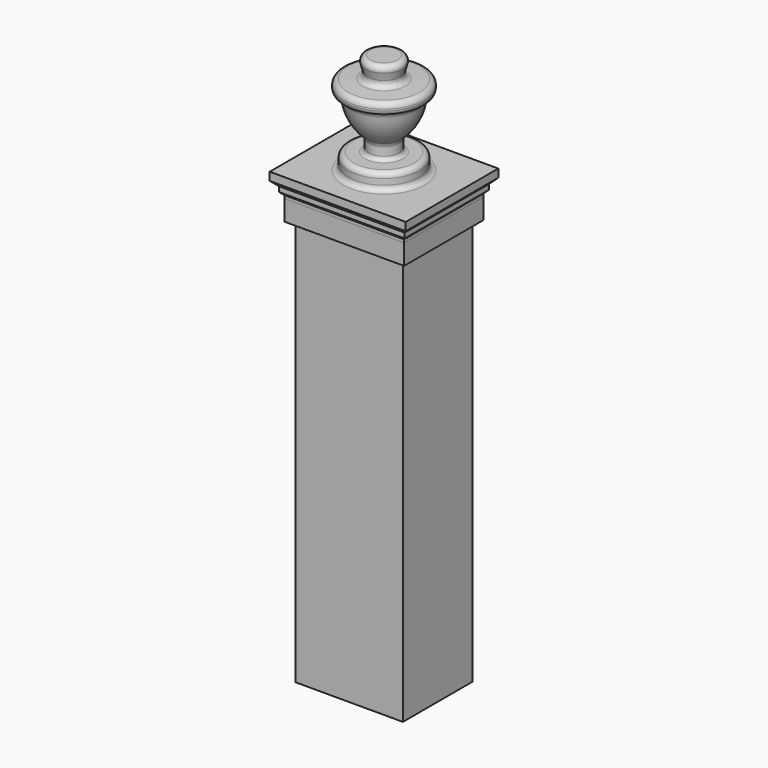
from build123d import *

# Parameters (mm, degrees)
F0_W     = 530
F0_H     = 430
F1_DEPTH = 2000
F2_W     = 590
F2_H     = 490
F3_DEPTH = 100
F6_W     = 510
F6_H     = 410
F7_DEPTH = 120
F10_R    = 25.4
F11_R    = 19.05


with BuildPart() as f1:
    # F0 (on Top) → F1 (new body)
    with BuildSketch(Plane.XY):
        Rectangle(F0_W, F0_H)
    extrude(amount=F1_DEPTH)

    # F2 (on face) → F3 (join)
    with BuildSketch(Plane.XY.offset(2000)):
        Rectangle(F2_W, F2_H)
    extrude(amount=F3_DEPTH)


with BuildPart() as f5:
    # F5: sweep along a path in F5_path
    with BuildLine(Plane(origin=(295, -245, 2100), x_dir=(0, 1, 0), z_dir=(0, 0, 1))) as f5_path:
        Line((0, 0), (0, 590))
        Line((0, 590), (490, 590))
        Line((490, 590), (490, 0))
        Line((490, 0), (0, 0))
    # F4 (on Right) → F5 (sweep)
    with BuildSketch(Plane.YZ):
        Polygon((-245, 2115), (-245, 2100), (-205, 2100), (-205, 2220), (-285, 2220), (-285, 2180), (-260, 2155), (-260, 2130), align=None)
    sweep(path=f5_path.line, transition=Transition.RIGHT)

    # F6 (on face) → F7 (join, through all)
    with BuildSketch(Plane.XY.offset(2220)):
        Rectangle(F6_W, F6_H)
    extrude(amount=-F7_DEPTH)

    # F8 (on Right) → F9 (revolve)
    with BuildSketch(Plane.YZ):
        with BuildLine():
            Line((100, 2720), (0, 2720))
            Line((0, 2720), (0, 2220))
            Line((0, 2220), (175, 2220))
            Line((175, 2220), (175, 2300))
            Line((175, 2300), (75, 2300))
            Line((75, 2300), (75, 2371.5957669105))
            ThreePointArc((75, 2371.5957669105), (139.8395872534, 2451.7615113993), (166.8133494995, 2551.2760069009))
            Line((166.8133494995, 2551.2760069009), (200, 2563.3549598581))
            Line((200, 2563.3549598581), (200, 2613.3549598581))
            Line((200, 2613.3549598581), (73.2050807569, 2620))
            Line((73.2050807569, 2620), (100, 2720))
        make_face()
    revolve(axis=Axis((0, 0, 1360), (0, 0, 1)))

    # F10
    f10_edges = [f5.edges().sort_by_distance(p)[0] for p in [
        (0, -175, 2220),
        (0, -175, 2300),
        (0, -75, 2371.595767),
        (0, -166.813349, 2551.276007),
        (0, -73.205081, 2620),
        (0, -200, 2563.35496),
        (0, -200, 2613.35496),
        (0, -100, 2720),
    ]]
    fillet(f10_edges, radius=F10_R)

    # F11
    f11_edges = [f5.edges().sort_by_distance(p)[0] for p in [
        (0, -75, 2300),
    ]]
    fillet(f11_edges, radius=F11_R)


solid = Compound([f1.part, f5.part])
